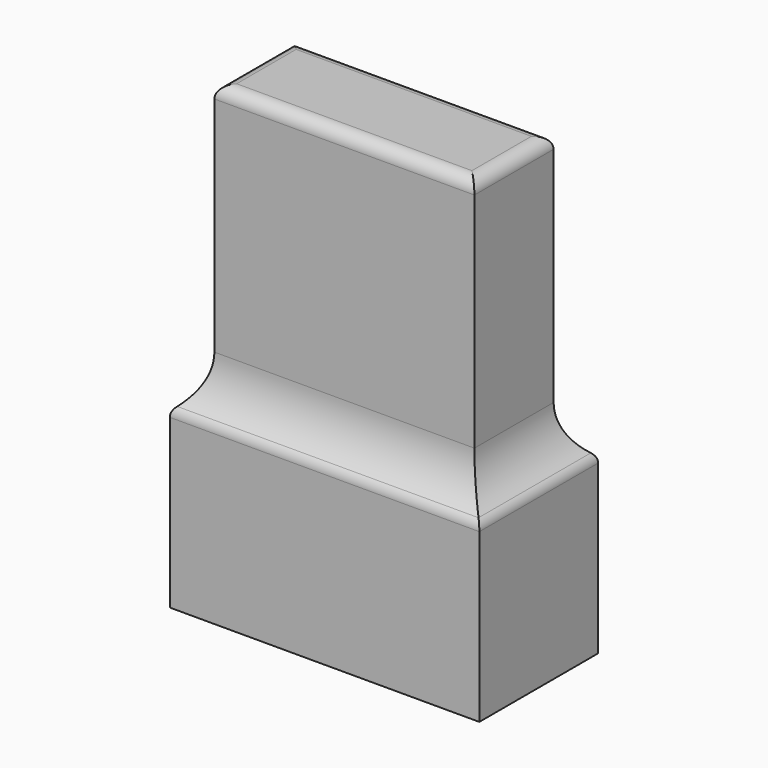
from build123d import *

# Parameters (mm, degrees)
F0_W           = 25
F0_H           = 12
F0_W_2         = 19
F0_H_2         = 8
F1_DEPTH       = 10
F2_W           = 21
F2_H           = 8
F2_W_2         = 17
F2_H_2         = 2
F3_DEPTH       = 25
F4_W           = 21
F4_H           = 8
F4_W_2         = 17
F4_H_2         = 2
F5_DEPTH       = 2
F6_W           = 25
F6_H           = 12
F7_DEPTH       = 4
F10_DEPTH      = 4
F10_DEPTH_BACK = 4
F11_T1_DEPTH   = 21
F11_T3_DEPTH   = 8
F11_T9_DEPTH   = 31
F11_T14_DEPTH  = 18
F11_T22_DEPTH  = 31
F11_T27_DEPTH  = 18
F11_T35_DEPTH  = 31
F11_T40_DEPTH  = 18
F11_T48_DEPTH  = 18
F11_T53_DEPTH  = 31
F12_R          = 1
F14_DEPTH      = 1


# Not quite as in the source:
# - a fillet or chamfer that OpenCascade refuses, or shapes differently, is made with other operations: its cross-section is extruded or revolved along the edge and cut away or added


with BuildPart() as f1:
    # F0 (on Top) → F1 (new body)
    with BuildSketch(Plane.XY):
        with Locations((12.5, 6)):
            Rectangle(F0_W, F0_H)
        with Locations((12.5, 6)):
            Rectangle(F0_W_2, F0_H_2, mode=Mode.SUBTRACT)
    extrude(amount=-F1_DEPTH)

    # F2 (on Top) → F3 (join)
    with BuildSketch(Plane.XY):
        with Locations((12.5, 6)):
            Rectangle(F2_W, F2_H)
        with Locations((12.5, 6)):
            Rectangle(F2_W_2, F2_H_2, mode=Mode.SUBTRACT)
    extrude(amount=F3_DEPTH)

    # F4 (on face) → F5 (join)
    with BuildSketch(Plane.XY.offset(25)):
        with Locations((12.5, 6)):
            Rectangle(F4_W, F4_H)
        with Locations((12.5, 6)):
            Rectangle(F4_W_2, F4_H_2, mode=Mode.SUBTRACT)
        with Locations((12.5, 6)):
            Rectangle(F4_W_2, F4_H_2)
    extrude(amount=F5_DEPTH)

    # F6 (on face) → F7 (join)
    with BuildSketch(Plane.XY):
        with Locations((12.5, 6)):
            Rectangle(F6_W, F6_H)
        Polygon((23, 2), (22, 2), (3, 2), (2, 2), (2, 10), (3, 10), (22, 10), (23, 10), align=None, mode=Mode.SUBTRACT)
    extrude(amount=F7_DEPTH)

    # F9 (on offset) → F10 (join, two sides)
    with BuildSketch(Plane.XZ.offset(-6)) as f10_sk:
        with BuildLine():
            Line((3, -7), (3, -8.5))
            Line((3, -8.5), (3.4671572875, -8.0328427125))
            ThreePointArc((3.4671572875, -8.0328427125), (3.5843145751, -7.75), (3.4671572875, -7.4671572875))
            Line((3.4671572875, -7.4671572875), (3, -7))
        make_face()
        with BuildLine():
            Line((21.5328427125, -8.0328427125), (22, -8.5))
            Line((22, -8.5), (22, -7))
            Line((22, -7), (21.5328427125, -7.4671572875))
            ThreePointArc((21.5328427125, -7.4671572875), (21.4156854249, -7.75), (21.5328427125, -8.0328427125))
        make_face()
    extrude(amount=F10_DEPTH)
    extrude(f10_sk.sketch, amount=-F10_DEPTH_BACK)

    # F11: fillet of radius 5 on 4 edges, made by hand

    # F11_s2 → F11_t1 (join)
    with BuildSketch(Plane.YZ.offset(2)):
        with BuildLine():
            ThreePointArc((0, 4), (1.472135955, 5.7639320225), (2, 8))
            Line((2, 8), (2, 4))
            Line((2, 4), (0, 4))
        make_face()
        with BuildLine():
            ThreePointArc((12, 4), (10.527864045, 5.7639320225), (10, 8))
            Line((10, 8), (10, 4))
            Line((10, 4), (12, 4))
        make_face()
    extrude(amount=F11_T1_DEPTH)

    # F11_s4 → F11_t3 (join)
    with BuildSketch(Plane.XZ.offset(-10)):
        with BuildLine():
            ThreePointArc((25, 4), (23.527864045, 5.7639320225), (23, 8))
            Line((23, 8), (23, 4))
            Line((23, 4), (25, 4))
        make_face()
        with BuildLine():
            ThreePointArc((0, 4), (1.472135955, 5.7639320225), (2, 8))
            Line((2, 8), (2, 4))
            Line((2, 4), (0, 4))
        make_face()
    extrude(amount=F11_T3_DEPTH)


with BuildPart() as f11_tool7:
    # F11_s8 → F11_t9 (new body)
    with BuildSketch(Plane.YZ.offset(-8)):
        with BuildLine():
            ThreePointArc((0, 4), (1.472135955, 5.7639320225), (2, 8))
            Line((2, 8), (2, 4))
            Line((2, 4), (0, 4))
        make_face()
    extrude(amount=F11_T9_DEPTH)

    split(bisect_by=Plane.YZ, keep=Keep.TOP)

    split(bisect_by=Plane.YZ.offset(2), keep=Keep.BOTTOM)


with BuildPart() as f11_tool12:
    # F11_s13 → F11_t14 (new body)
    with BuildSketch(Plane.XZ.offset(8)):
        with BuildLine():
            ThreePointArc((0, 4), (1.472135955, 5.7639320225), (2, 8))
            Line((2, 8), (2, 4))
            Line((2, 4), (0, 4))
        make_face()
    extrude(amount=-F11_T14_DEPTH)

    split(bisect_by=Plane.XZ, keep=Keep.BOTTOM)

    split(bisect_by=Plane.XZ.offset(-2), keep=Keep.TOP)


with BuildPart() as f11_tool7_1:
    add(f11_tool7.part)

    # F11_t17: intersect F11_tool12
    add(f11_tool12.part, mode=Mode.INTERSECT)


with BuildPart() as f1_1:
    add(f1.part)

    # F11_t5: union F11_tool7
    add(f11_tool7_1.part)


with BuildPart() as f11_tool20:
    # F11_s21 → F11_t22 (new body)
    with BuildSketch(Plane.YZ.offset(2)):
        with BuildLine():
            ThreePointArc((0, 4), (1.472135955, 5.7639320225), (2, 8))
            Line((2, 8), (2, 4))
            Line((2, 4), (0, 4))
        make_face()
    extrude(amount=F11_T22_DEPTH)

    split(bisect_by=Plane.YZ.offset(25), keep=Keep.BOTTOM)

    split(bisect_by=Plane.YZ.offset(23), keep=Keep.TOP)


with BuildPart() as f11_tool25:
    # F11_s26 → F11_t27 (new body)
    with BuildSketch(Plane.XZ.offset(-10)):
        with BuildLine():
            ThreePointArc((25, 4), (23.527864045, 5.7639320225), (23, 8))
            Line((23, 8), (23, 4))
            Line((23, 4), (25, 4))
        make_face()
    extrude(amount=F11_T27_DEPTH)

    split(bisect_by=Plane.XZ, keep=Keep.BOTTOM)

    split(bisect_by=Plane.XZ.offset(-2), keep=Keep.TOP)


with BuildPart() as f11_tool20_1:
    add(f11_tool20.part)

    # F11_t30: intersect F11_tool25
    add(f11_tool25.part, mode=Mode.INTERSECT)


with BuildPart() as f1_2:
    add(f1_1.part)

    # F11_t18: union F11_tool20
    add(f11_tool20_1.part)


with BuildPart() as f11_tool33:
    # F11_s34 → F11_t35 (new body)
    with BuildSketch(Plane.YZ.offset(33)):
        with BuildLine():
            ThreePointArc((12, 4), (10.527864045, 5.7639320225), (10, 8))
            Line((10, 8), (10, 4))
            Line((10, 4), (12, 4))
        make_face()
    extrude(amount=-F11_T35_DEPTH)

    split(bisect_by=Plane.YZ.offset(25), keep=Keep.BOTTOM)

    split(bisect_by=Plane.YZ.offset(23), keep=Keep.TOP)


with BuildPart() as f11_tool38:
    # F11_s39 → F11_t40 (new body)
    with BuildSketch(Plane.XZ.offset(-20)):
        with BuildLine():
            ThreePointArc((25, 4), (23.527864045, 5.7639320225), (23, 8))
            Line((23, 8), (23, 4))
            Line((23, 4), (25, 4))
        make_face()
    extrude(amount=F11_T40_DEPTH)

    split(bisect_by=Plane.XZ.offset(-12), keep=Keep.TOP)

    split(bisect_by=Plane.XZ.offset(-10), keep=Keep.BOTTOM)


with BuildPart() as f11_tool33_1:
    add(f11_tool33.part)

    # F11_t43: intersect F11_tool38
    add(f11_tool38.part, mode=Mode.INTERSECT)


with BuildPart() as f1_3:
    add(f1_2.part)

    # F11_t31: union F11_tool33
    add(f11_tool33_1.part)


with BuildPart() as f11_tool46:
    # F11_s47 → F11_t48 (new body)
    with BuildSketch(Plane.XZ.offset(-2)):
        with BuildLine():
            ThreePointArc((0, 4), (1.472135955, 5.7639320225), (2, 8))
            Line((2, 8), (2, 4))
            Line((2, 4), (0, 4))
        make_face()
    extrude(amount=-F11_T48_DEPTH)

    split(bisect_by=Plane.XZ.offset(-12), keep=Keep.TOP)

    split(bisect_by=Plane.XZ.offset(-10), keep=Keep.BOTTOM)


with BuildPart() as f11_tool51:
    # F11_s52 → F11_t53 (new body)
    with BuildSketch(Plane.YZ.offset(23)):
        with BuildLine():
            ThreePointArc((12, 4), (10.527864045, 5.7639320225), (10, 8))
            Line((10, 8), (10, 4))
            Line((10, 4), (12, 4))
        make_face()
    extrude(amount=-F11_T53_DEPTH)

    split(bisect_by=Plane.YZ, keep=Keep.TOP)

    split(bisect_by=Plane.YZ.offset(2), keep=Keep.BOTTOM)


with BuildPart() as f11_tool46_1:
    add(f11_tool46.part)

    # F11_t56: intersect F11_tool51
    add(f11_tool51.part, mode=Mode.INTERSECT)


with BuildPart() as f1_4:
    add(f1_3.part)

    # F11_t44: union F11_tool46
    add(f11_tool46_1.part)

    # F12
    f12_edges = [f1_4.edges().sort_by_distance(p)[0] for p in [
        (23, 6, 27),
        (12.5, 2, 27),
        (2, 6, 27),
        (12.5, 10, 27),
        (12.5, 12, 4),
        (25, 6, 4),
        (12.5, 0, 4),
        (0, 6, 4),
    ]]
    fillet(f12_edges, radius=F12_R)

    # F13 (on face) → F14 (cut)
    with BuildSketch(Plane(origin=(0, 10, 0), x_dir=(-1, 0, 0), z_dir=(0, 1, 0))):
        Polygon((-12.5, 20.9), (-17, 13.1057713659), (-8, 13.1057713659), align=None)
        Polygon((-16.1339745962, 13.6057713659), (-14.4613248654, 16.502885683), (-12.7886751346, 13.6057713659), align=None, mode=Mode.SUBTRACT)
        Polygon((-12.5, 13.6057713659), (-14.3169872981, 16.752885683), (-10.6830127019, 16.752885683), align=None, mode=Mode.SUBTRACT)
        Polygon((-8.8660254038, 13.6057713659), (-12.2113248654, 13.6057713659), (-10.5386751346, 16.502885683), align=None, mode=Mode.SUBTRACT)
        Polygon((-12.5, 19.9), (-10.8273502692, 17.002885683), (-14.1726497308, 17.002885683), align=None, mode=Mode.SUBTRACT)
    extrude(amount=-F14_DEPTH, mode=Mode.SUBTRACT)


solid = f1_4.part
